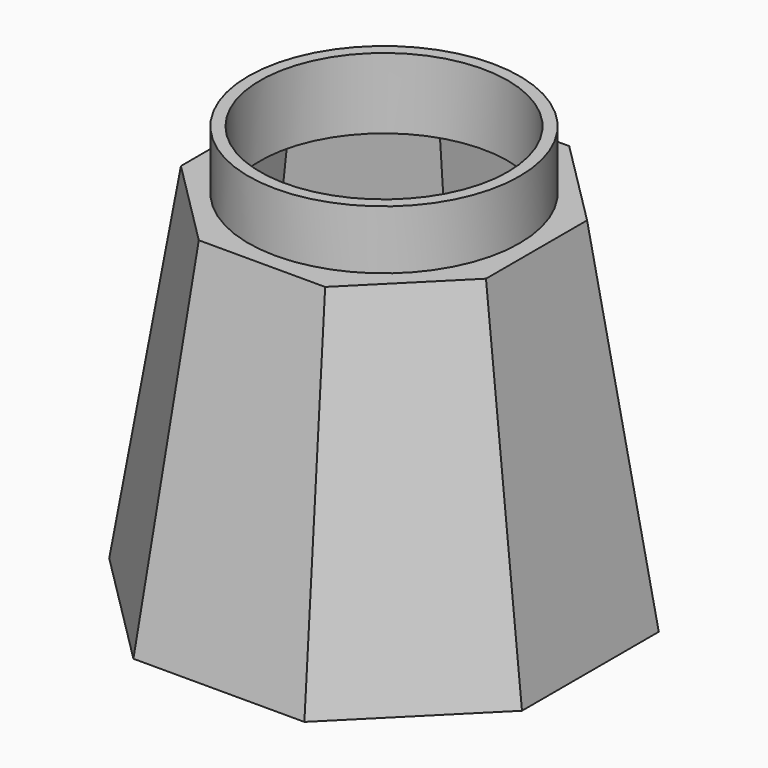
from build123d import *

# Parameters (mm, degrees)
F4_R     = 29.21
F5_DEPTH = 12.7
F6_T     = -2.54


with BuildPart() as f3:
    # F0 (on Top) → F3 section 0
    with BuildSketch(Plane.XY):
        Polygon((18.4117928475, 44.45), (-18.4117928475, 44.45), (-44.45, 18.4117928475), (-44.45, -18.4117928475), (-18.4117928475, -44.45), (18.4117928475, -44.45), (44.45, -18.4117928475), (44.45, 18.4117928475), align=None)
    # F2 (on offset) → F3 section 1
    with BuildSketch(Plane.XY.offset(76.2)):
        Polygon((32.8531561761, -13.6082228549), (32.8531561761, 13.6082228549), (13.6082228549, 32.8531561761), (-13.6082228549, 32.8531561761), (-32.8531561761, 13.6082228549), (-32.8531561761, -13.6082228549), (-13.6082228549, -32.8531561761), (13.6082228549, -32.8531561761), align=None)
    loft()

    # F4 (on face) → F5 (join)
    with BuildSketch(Plane.XY.offset(76.2)):
        Circle(F4_R)
    extrude(amount=F5_DEPTH)

    # F6
    f6_openings = [f3.faces().sort_by_distance(p)[0] for p in [
        (0, 0, 88.9),
    ]]
    offset(amount=F6_T, openings=f6_openings, kind=Kind.INTERSECTION)


solid = f3.part
